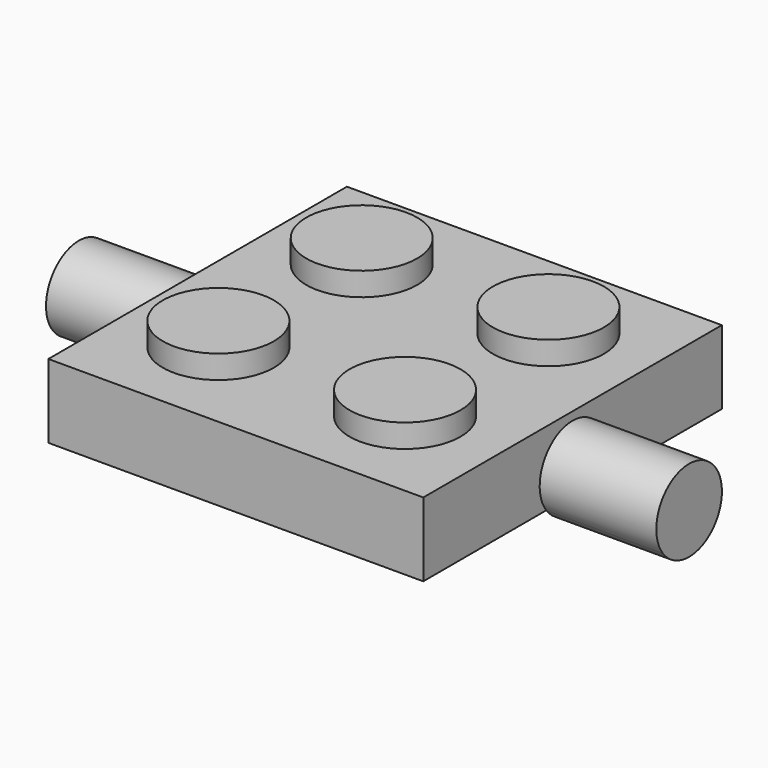
from build123d import *

# Parameters (mm, degrees)
F0_W     = 16.0737466067
F0_H     = 3.1658632215
F1_DEPTH = 16
F2_R     = 2.3801305446
F2_R_2   = 2.3799092656
F2_R_3   = 2.3780181716
F2_R_4   = 2.3779678295
F3_DEPTH = 1
F5_DEPTH = 5
F6_R     = 1.7583787775
F7_DEPTH = 5


with BuildPart() as f1:
    # F0 (on Front) → F1 (new body)
    with BuildSketch(Plane.XZ):
        with Locations((8.0368733034, 1.5829316108)):
            Rectangle(F0_W, F0_H)
    extrude(amount=F1_DEPTH)

    # F2 (on face) → F3 (join)
    with BuildSketch(Plane.XY.offset(3.1658632215)):
        with Locations((3.9132172242, -11.7802852765)):
            Circle(F2_R)
        with Locations((11.9156921282, -11.7802852765)):
            Circle(F2_R_2)
        with Locations((11.9156921282, -4.0964945219)):
            Circle(F2_R_3)
        with Locations((3.9132172242, -4.0964945219)):
            Circle(F2_R_4)
    extrude(amount=F3_DEPTH)

    # F4 (on face) → F5 (join)
    with BuildSketch(Plane.YZ.offset(16.0737466067)):
        with BuildLine():
            ThreePointArc((-6.5959664397, 0), (-6.3346840784, 0.4988617172), (-6.2445068398, 1.0547389975))
            ThreePointArc((-6.2445068398, 1.0547389975), (-8.5587628976, 2.7229405364), (-9.409804795, 0))
            ThreePointArc((-9.409804795, 0), (-8.0028856173, -0.70363978), (-6.5959664397, 0))
        make_face()
    extrude(amount=F5_DEPTH)

    # F6 (on Right) → F7 (join)
    with BuildSketch(Plane.YZ):
        with Locations((-8.1170331687, 1.0434978176)):
            Circle(F6_R)
    extrude(amount=-F7_DEPTH)


solid = f1.part
